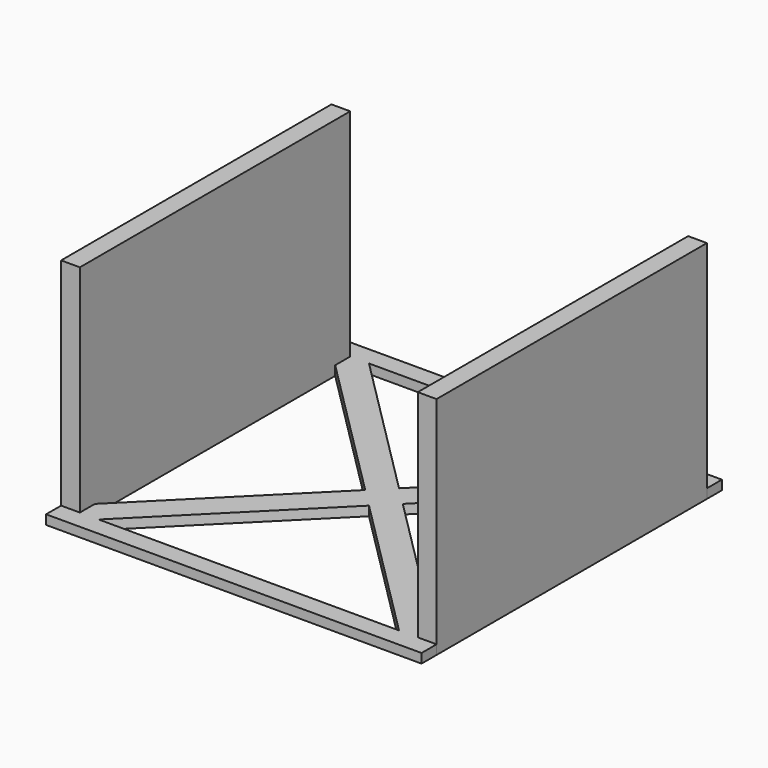
from build123d import *

# Parameters (mm, degrees)
F0_W     = 6.35
F0_H     = 6.35
F1_DEPTH = 3.175
F2_DEPTH = 76.2
F3_DEPTH = 76.2


with BuildPart() as f1:
    # F0 (on Top) → F1 (new body)
    with BuildSketch(Plane.XY):
        with Locations((-90.4763010761, -75.1771691605)):
            Rectangle(F0_W, F0_H)
        Polygon((-42.8513010761, -21.2021691605), (-93.6513010761, -72.0021691605), (-87.3013010761, -72.0021691605), (-87.3013010761, -78.3521691605), (-36.5013010761, -27.5521691605), align=None)
        Polygon((20.6486989239, -72.0021691605), (-30.1513010761, -21.2021691605), (-36.5013010761, -27.5521691605), (14.2986989239, -78.3521691605), (14.2986989239, -72.0021691605), align=None)
        Polygon((-36.5013010761, -14.8521691605), (-87.3013010761, 35.9478308395), (-87.3013010761, 29.5978308395), (-93.6439880831, 29.5978308395), (-93.6439796514, 29.5905094148), (-42.8513010761, -21.2021691605), align=None)
        Polygon((14.2986989239, 29.5978308395), (14.2986989239, 35.9478308395), (-36.5013010761, -14.8521691605), (-30.1513010761, -21.2021691605), (20.6486989239, 29.5978308395), align=None)
        with Locations((17.4736989239, 32.7728308395)):
            Rectangle(F0_W, F0_H)
        Polygon((-30.1513010761, -21.2021691605), (-36.5013010761, -14.8521691605), (-42.8513010761, -21.2021691605), (-36.5013010761, -27.5521691605), align=None)
        Polygon((-87.3013010761, 35.9478308395), (-93.6513010761, 35.9478308395), (-93.6439880831, 29.5978308395), (-87.3013010761, 29.5978308395), align=None)
        with Locations((17.4736989239, -75.1771691605)):
            Rectangle(F0_W, F0_H)
        Polygon((-100.0013010761, 35.9478308395), (-93.6513010761, 35.9478308395), (-87.3013010761, 35.9478308395), (14.2986989239, 35.9478308395), (20.6486989239, 35.9478308395), (26.9986989239, 35.9478308395), (26.9986989239, 42.2978308395), (-100.0013010761, 42.2978308395), align=None)
        Polygon((-93.6513010761, -78.3521691605), (-100.0013010761, -78.3521691605), (-100.0013010761, -84.7021691605), (26.9986989239, -84.7021691605), (26.9986989239, -78.3521691605), (20.6486989239, -78.3521691605), (14.2986989239, -78.3521691605), (4.1404153609, -78.3521691605), (-87.3013010761, -78.3521691605), align=None)
    extrude(amount=F1_DEPTH)


with BuildPart() as f2:
    # F0 (on Top) → F2 (new body)
    with BuildSketch(Plane.XY):
        Polygon((-93.6513010761, 29.5978308395), (-93.6513010761, 35.9478308395), (-100.0013010761, 35.9478308395), (-100.0013010761, -78.3521691605), (-93.6513010761, -78.3521691605), (-93.6513010761, -72.0021691605), align=None)
    extrude(amount=F2_DEPTH)


with BuildPart() as f3:
    # F0 (on Top) → F3 (new body)
    with BuildSketch(Plane.XY):
        Polygon((26.9986989239, 35.9478308395), (20.6486989239, 35.9478308395), (20.6486989239, 29.5978308395), (20.6486989239, -72.0021691605), (20.6486989239, -78.3521691605), (26.9986989239, -78.3521691605), align=None)
    extrude(amount=F3_DEPTH)


solid = Compound([f1.part, f2.part, f3.part])
